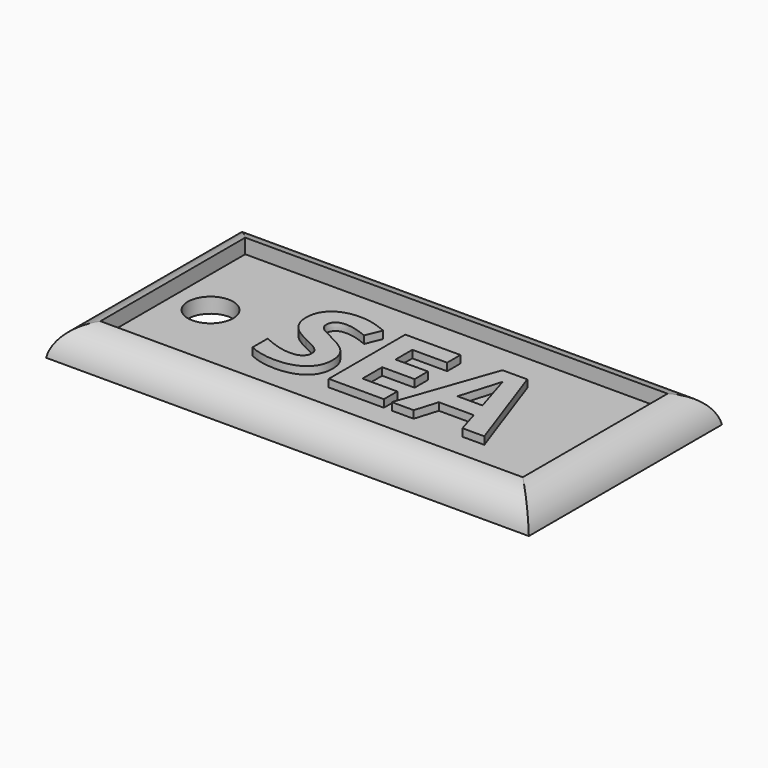
from build123d import *

# Parameters (mm, degrees)
F0_W         = 44.45
F0_H         = 19.05
F0_R         = 2.38125
F1_DEPTH     = 1.5875
F0_W_2       = 50.8
F0_H_2       = 25.4
F2_DEPTH     = 3.175
F3_TEXT_SIZE = 14.1111111111
F5_DEPTH     = 0.79375
F6_T1_DEPTH  = 69.5835533113
F6_T3_DEPTH  = 44.1835533113


# Not quite as in the source:
# - a fillet or chamfer that OpenCascade refuses, or shapes differently, is made with other operations: its cross-section is extruded or revolved along the edge and cut away or added
# - Text() gives the source's letters only with a copy of the font that has no kerning and outlines rounded to 1/6400 em; it was checked with that copy


with BuildPart() as f1:
    # F0 (on Top) → F1 (new body)
    with BuildSketch(Plane.XY):
        with Locations((25.4, 12.7)):
            Rectangle(F0_W, F0_H)
        with Locations((7.14375, 12.7)):
            Circle(F0_R, mode=Mode.SUBTRACT)
    extrude(amount=F1_DEPTH)

    # F0 (on Top) → F2 (join)
    with BuildSketch(Plane.XY):
        with Locations((25.4, 12.7)):
            Rectangle(F0_W_2, F0_H_2)
        with Locations((25.4, 12.7)):
            Rectangle(F0_W, F0_H, mode=Mode.SUBTRACT)
    extrude(amount=F2_DEPTH)

    # F3 (on face) → F5 (join)
    with BuildSketch(Plane.XY.offset(1.5875)):
        with Locations((14.2937937918, 8.0129120697)):
            Text('SEA', F3_TEXT_SIZE, font='Open Sans', font_style=FontStyle.BOLD, text_align=(TextAlign.LEFT, TextAlign.BOTTOM))
    extrude(amount=F5_DEPTH)

    # F6: fillet of radius 3.81 on 4 edges, made by hand

    # F6_s2 → F6_t1 (cut)
    with BuildSketch(Plane.YZ.offset(-9.3917766557)):
        with BuildLine():
            ThreePointArc((0, 0), (1.2973662374, 2.2749355663), (3.7567106623, 3.175))
            Line((3.7567106623, 3.175), (0, 3.175))
            Line((0, 3.175), (0, 0))
        make_face()
        with BuildLine():
            ThreePointArc((25.4, 0), (24.1026337626, 2.2749355663), (21.6432893377, 3.175))
            Line((21.6432893377, 3.175), (25.4, 3.175))
            Line((25.4, 3.175), (25.4, 0))
        make_face()
    extrude(amount=F6_T1_DEPTH, mode=Mode.SUBTRACT)

    # F6_s4 → F6_t3 (cut)
    with BuildSketch(Plane.XZ.offset(-34.7917766557)):
        with BuildLine():
            ThreePointArc((0, 0), (1.2973662374, 2.2749355663), (3.7567106623, 3.175))
            Line((3.7567106623, 3.175), (0, 3.175))
            Line((0, 3.175), (0, 0))
        make_face()
        with BuildLine():
            ThreePointArc((50.8, 0), (49.5026337626, 2.2749355663), (47.0432893377, 3.175))
            Line((47.0432893377, 3.175), (50.8, 3.175))
            Line((50.8, 3.175), (50.8, 0))
        make_face()
    extrude(amount=F6_T3_DEPTH, mode=Mode.SUBTRACT)


solid = f1.part
